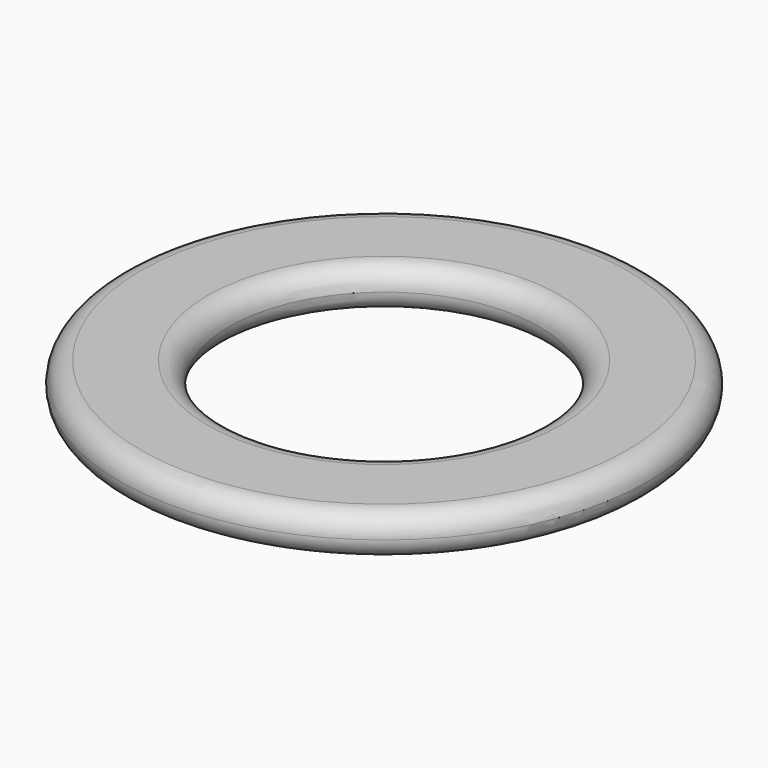
from build123d import *

# Parameters (mm, degrees)
F0_R     = 12.72999994
F0_R_2   = 7.5
F1_DEPTH = 2
F2_R     = 0.99999
F3_R     = 0.99999


# Not quite as in the source:
# - a fillet or chamfer is up to 0.001 mm smaller than in the source, because OpenCascade refuses the exact size


with BuildPart() as f1:
    # F0 (on Top) → F1 (new body)
    with BuildSketch(Plane.XY):
        Circle(F0_R)
        Circle(F0_R_2, mode=Mode.SUBTRACT)
    extrude(amount=F1_DEPTH)

    # F2 (radius 1 in the source; OpenCascade refuses exactly that, so slightly less here)
    f2_edges = [f1.edges().sort_by_distance(p)[0] for p in [
        (12.73, 0, 1),
        (-12.73, 0, 0),
        (-12.73, 0, 2),
    ]]
    fillet(f2_edges, radius=F2_R)

    # F3 (radius 1 in the source; OpenCascade refuses exactly that, so slightly less here)
    f3_edges = [f1.edges().sort_by_distance(p)[0] for p in [
        (7.5, 0, 1),
        (-7.5, 0, 0),
        (-7.5, 0, 2),
    ]]
    fillet(f3_edges, radius=F3_R)


solid = f1.part
